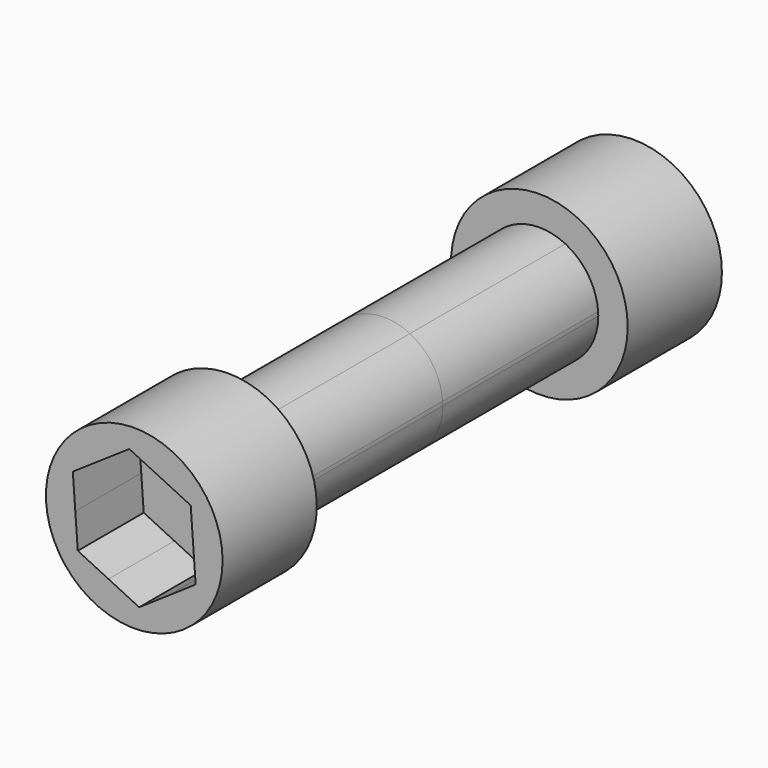
from build123d import *

# Parameters (mm, degrees)
F1_DEPTH = 2.0955
F0_R     = 0.9525
F2_DEPTH = 0.381
F3_R     = 0.9525
F4_DEPTH = 0.889


with BuildPart() as f1:
    # F0 (on Front) → F1 (new body)
    with BuildSketch(Plane.XZ):
        with BuildLine():
            ThreePointArc((-50.4787408751, 29.4385525432), (-50.27185395, 29.6671320557), (-50.1970108056, 29.9662128091))
            ThreePointArc((-50.1970108056, 29.9662128091), (-50.1973603622, 29.9872797188), (-50.1984086471, 30.0083234346))
            ThreePointArc((-50.1984086471, 30.0083234346), (-50.3043505199, 30.31948271), (-50.5516784903, 30.5359836341))
            ThreePointArc((-50.5516784903, 30.5359836341), (-50.8741213768, 30.5998149712), (-51.1852807654, 30.4938730554))
            ThreePointArc((-51.1852807654, 30.4938730554), (-51.4017816859, 30.246545012), (-51.4656129641, 29.9241021836))
            ThreePointArc((-51.4656129641, 29.9241021836), (-51.3596710927, 29.6129429103), (-51.1123431255, 29.3964419864))
            ThreePointArc((-51.1123431255, 29.3964419864), (-50.7899002546, 29.3326106457), (-50.4787408751, 29.4385525432))
        make_face()
    extrude(amount=-F1_DEPTH)

    # F0 (on Front) → F2 (join)
    with BuildSketch(Plane.XZ):
        with Locations((-50.8320108056, 29.9662128091)):
            Circle(F0_R)
        Polygon((-50.2227212209, 30.3741338006), (-50.1984086471, 30.0083234346), (-50.1740960719, 29.6425130463), (-50.4787408751, 29.4385525432), (-50.7833856565, 29.2345920547), (-51.1123431255, 29.3964419864), (-51.4413003903, 29.5582918175), (-51.4656129641, 29.9241021836), (-51.4899255394, 30.2899125719), (-51.1852807654, 30.4938730554), (-50.8806359547, 30.6978335634), (-50.5516784903, 30.5359836341), align=None, mode=Mode.SUBTRACT)
        with BuildLine():
            ThreePointArc((-50.4787408751, 29.4385525432), (-50.27185395, 29.6671320557), (-50.1970108056, 29.9662128091))
            ThreePointArc((-50.1970108056, 29.9662128091), (-50.1973603622, 29.9872797188), (-50.1984086471, 30.0083234346))
            ThreePointArc((-50.1984086471, 30.0083234346), (-50.3043505199, 30.31948271), (-50.5516784903, 30.5359836341))
            ThreePointArc((-50.5516784903, 30.5359836341), (-50.8741213768, 30.5998149712), (-51.1852807654, 30.4938730554))
            ThreePointArc((-51.1852807654, 30.4938730554), (-51.4017816859, 30.246545012), (-51.4656129641, 29.9241021836))
            ThreePointArc((-51.4656129641, 29.9241021836), (-51.3596710927, 29.6129429103), (-51.1123431255, 29.3964419864))
            ThreePointArc((-51.1123431255, 29.3964419864), (-50.7899002546, 29.3326106457), (-50.4787408751, 29.4385525432))
        make_face()
        with BuildLine():
            ThreePointArc((-50.1984086471, 30.0083234346), (-50.1973603622, 29.9872797188), (-50.1970108056, 29.9662128091))
            ThreePointArc((-50.1970108056, 29.9662128091), (-50.27185395, 29.6671320557), (-50.4787408751, 29.4385525432))
            Line((-50.4787408751, 29.4385525432), (-50.1740960719, 29.6425130463))
            Line((-50.1740960719, 29.6425130463), (-50.1984086471, 30.0083234346))
        make_face()
        with BuildLine():
            ThreePointArc((-50.5516784903, 30.5359836341), (-50.3043505199, 30.31948271), (-50.1984086471, 30.0083234346))
            Line((-50.1984086471, 30.0083234346), (-50.2227212209, 30.3741338006))
            Line((-50.2227212209, 30.3741338006), (-50.5516784903, 30.5359836341))
        make_face()
        with BuildLine():
            Line((-50.7833856565, 29.2345920547), (-50.4787408751, 29.4385525432))
            ThreePointArc((-50.4787408751, 29.4385525432), (-50.7899002546, 29.3326106457), (-51.1123431255, 29.3964419864))
            Line((-51.1123431255, 29.3964419864), (-50.7833856565, 29.2345920547))
        make_face()
        with BuildLine():
            ThreePointArc((-51.1852807654, 30.4938730554), (-50.8741213768, 30.5998149712), (-50.5516784903, 30.5359836341))
            Line((-50.5516784903, 30.5359836341), (-50.8806359547, 30.6978335634))
            Line((-50.8806359547, 30.6978335634), (-51.1852807654, 30.4938730554))
        make_face()
        with BuildLine():
            Line((-51.4413003903, 29.5582918175), (-51.1123431255, 29.3964419864))
            ThreePointArc((-51.1123431255, 29.3964419864), (-51.3596710927, 29.6129429103), (-51.4656129641, 29.9241021836))
            Line((-51.4656129641, 29.9241021836), (-51.4413003903, 29.5582918175))
        make_face()
        with BuildLine():
            ThreePointArc((-51.4656129641, 29.9241021836), (-51.4017816859, 30.246545012), (-51.1852807654, 30.4938730554))
            Line((-51.1852807654, 30.4938730554), (-51.4899255394, 30.2899125719))
            Line((-51.4899255394, 30.2899125719), (-51.4656129641, 29.9241021836))
        make_face()
    extrude(amount=F2_DEPTH)

    # F3 (on face) → F4 (join)
    with BuildSketch(Plane.XZ.offset(0.381)):
        with Locations((-50.8320108056, 29.9662128091)):
            Circle(F3_R)
        Polygon((-50.2231179997, 30.3795862702), (-50.1963452388, 30.012584543), (-50.1695724841, 29.6455829016), (-50.4740186105, 29.4388963588), (-50.77846529, 29.2322094405), (-51.1096844946, 29.3925244155), (-51.4409036115, 29.552839348), (-51.4676763724, 29.9198410751), (-51.4944491271, 30.2868427166), (-51.1900030005, 30.4935292595), (-50.8855563212, 30.7002161777), (-50.5543371681, 30.5399012276), align=None, mode=Mode.SUBTRACT)
    extrude(amount=F4_DEPTH)

    # F5: F1 across face


with BuildPart() as f1_1:
    add(f1.part)
    add(f1.part.mirror(Plane(origin=(-50.8320108056, 2.0955, 29.9662128091), x_dir=(1, 0, 0), z_dir=(0, 1, 0))))


solid = f1_1.part
